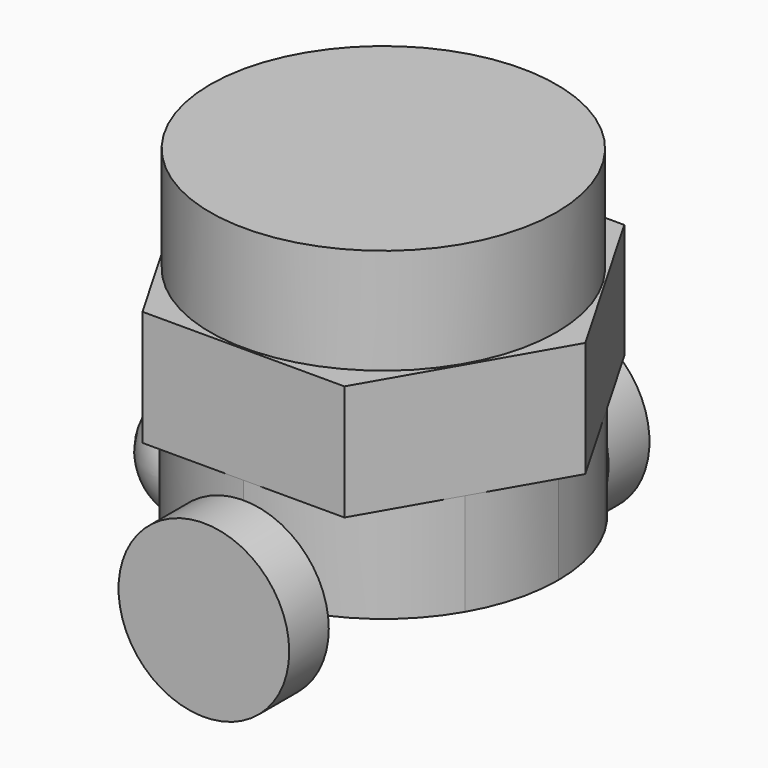
from build123d import *

# Parameters (mm, degrees)
F0_R     = 26.671348359
F1_DEPTH = 16.256
F3_DEPTH = 17.78
F5_DEPTH = 15.748
F6_R     = 13.1367039981
F7_DEPTH = 7.874
F8_R     = 13.144903068
F9_DEPTH = 7.62


# Not quite as in the source:
# - the program builds the solid bodies; features that only make, move or delete a surface that nothing else refers to are left out


with BuildPart() as f1:
    # F0 (on Top) → F1 (new body)
    with BuildSketch(Plane.XY):
        Circle(F0_R)
    extrude(amount=F1_DEPTH)

    # F2 (on Top) → F3 (join)
    with BuildSketch(Plane.XY):
        Polygon((15.5526856108, 26.9380416721), (-15.5526856108, 26.9380416721), (-31.1053712217, 0), (-15.5526856108, -26.9380416721), (15.5526856108, -26.9380416721), (31.1053712217, 0), align=None)
    extrude(amount=-F3_DEPTH)

    # F4 (on face) → F5 (join)
    with BuildSketch(Plane(origin=(0, 0, -17.78), x_dir=(1, 0, 0), z_dir=(0, 0, -1))):
        with BuildLine():
            ThreePointArc((23.3290284987, -13.4690206932), (26.0201501821, -6.9720781429), (26.9380416721, 0))
            ThreePointArc((26.9380416721, 0), (26.0201501337, 6.9720783236), (23.3290283116, 13.4690210173))
            ThreePointArc((23.3290283116, 13.4690210173), (13.4690207454, 23.3290284686), (0, 26.9380416721))
            ThreePointArc((0, 26.9380416721), (-13.4690205688, 23.3290285706), (-23.3290281076, 13.4690213707))
            ThreePointArc((-23.3290281076, 13.4690213707), (-26.9380416721, 4.834e-07), (-23.329028591, -13.4690205333))
            ThreePointArc((-23.329028591, -13.4690205333), (-13.4690209874, -23.3290283289), (0, -26.9380416721))
            ThreePointArc((0, -26.9380416721), (13.4690209075, -23.329028375), (23.3290284987, -13.4690206932))
        make_face()
    extrude(amount=F5_DEPTH)

    # F12 (on face) → F13 (revolve)
    with BuildSketch(Plane(origin=(0, 0, -33.528), x_dir=(1, 0, 0), z_dir=(0, 0, -1))):
        with BuildLine():
            Line((-26.9380416721, 1.35e-08), (-26.9380416721, 8.9419854241))
            ThreePointArc((-26.9380416721, 8.9419854241), (-35.8800270962, 0), (-26.9380416721, -8.9419854241))
            Line((-26.9380416721, -8.9419854241), (-26.9380416721, 1.35e-08))
        make_face()
    revolve(axis=Axis((-26.9380416721, 0, -33.528), (0, 1, 0)))


with BuildPart() as f7:
    # F6 (on face) → F7 (new body)
    with BuildSketch(Plane(origin=(0, 26.9380416721, 0), x_dir=(-1, 0, 0), z_dir=(0, 1, 0))):
        with Locations((0, -33.3710052073)):
            Circle(F6_R)
    extrude(amount=F7_DEPTH)


with BuildPart() as f9:
    # F8 (on face) → F9 (new body)
    with BuildSketch(Plane.XZ.offset(26.9380416721)):
        with Locations((0, -33.6390472949)):
            Circle(F8_R)
    extrude(amount=F9_DEPTH)


solid = Compound([f1.part, f7.part, f9.part])
